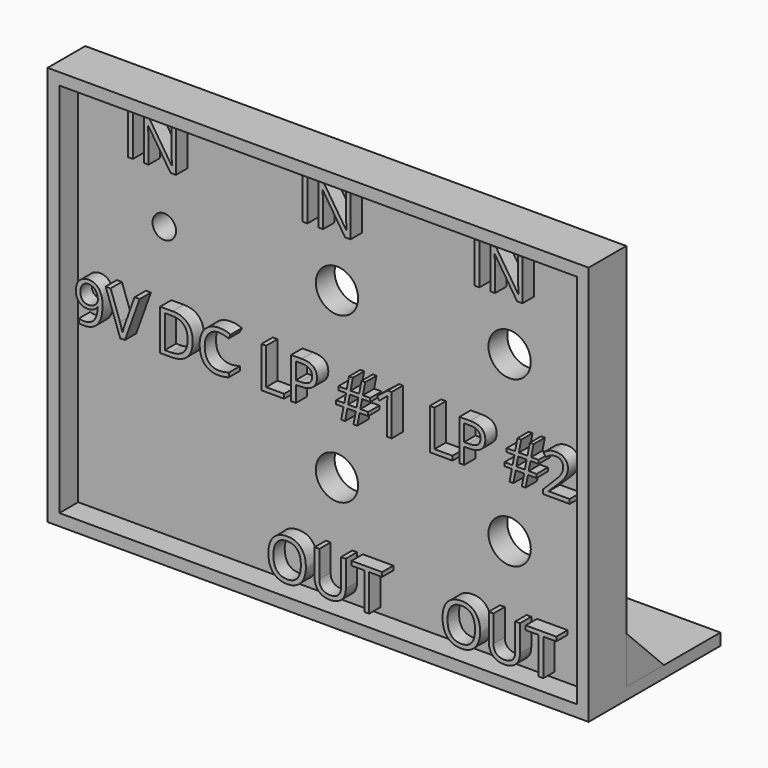
from build123d import *

# Parameters (mm, degrees)
F0_W          = 110
F0_H          = 80
F0_R          = 4.5
F0_R_2        = 2.5
F0_W_2        = 1.0082380031
F0_H_2        = 8.6754038348
F1_DEPTH      = 5
F2_DEPTH      = 10
F3_DEPTH      = 10
F3_DEPTH_BACK = 25
F0_TEXT_SIZE  = 12.1520211299
F4_DEPTH      = 8
F6_DEPTH      = 57.5


# Not quite as in the source:
# - Text() gives the source's letters only with a copy of the font that has no kerning and outlines rounded to 1/6400 em; it was checked with that copy


with BuildPart() as f1:
    # F0 (on Front) → F1 (new body)
    with BuildSketch(Plane.XZ):
        Rectangle(F0_W, F0_H)
        with BuildLine():
            add(Edge.make_bspline(
                [(-5.2528080414, -31.1302977692), (-4.2027974656, -32.3170185826), (-4.2027974656, -34.4056472143)],
                knots=[0, 0, 0, 1, 1, 1], degree=2))
            add(Edge.make_bspline(
                [(-4.2027974656, -34.4056472143), (-4.2027974656, -36.4885795861), (-5.256605548, -37.6819460362)],
                knots=[0, 0, 0, 1, 1, 1], degree=2))
            add(Edge.make_bspline(
                [(-5.256605548, -37.6819460362), (-6.3104136304, -38.8753124862), (-8.184483139, -38.8753124862)],
                knots=[0, 0, 0, 1, 1, 1], degree=2))
            add(Edge.make_bspline(
                [(-8.184483139, -38.8753124862), (-10.1003252203, -38.8753124862), (-11.1417914062, -37.7028323225)],
                knots=[0, 0, 0, 1, 1, 1], degree=2))
            add(Edge.make_bspline(
                [(-11.1417914062, -37.7028323225), (-12.1832575921, -36.5303521588), (-12.1832575921, -34.3942546945)],
                knots=[0, 0, 0, 1, 1, 1], degree=2))
            add(Edge.make_bspline(
                [(-12.1832575921, -34.3942546945), (-12.1832575921, -32.27524601), (-11.1389432762, -31.1094114829)],
                knots=[0, 0, 0, 1, 1, 1], degree=2))
            add(Edge.make_bspline(
                [(-11.1389432762, -31.1094114829), (-10.0946289604, -29.9435769557), (-8.1730906192, -29.9435769557)],
                knots=[0, 0, 0, 1, 1, 1], degree=2))
            add(Edge.make_bspline(
                [(-8.1730906192, -29.9435769557), (-6.3028186172, -29.9435769557), (-5.2528080414, -31.1302977692)],
                knots=[0, 0, 0, 1, 1, 1], degree=2))
        make_face(mode=Mode.SUBTRACT)
        with BuildLine():
            add(Edge.make_bspline(
                [(-47.7825725199, 2.592958442), (-47.4265562758, 1.7242788066), (-47.4265562758, 0.543254253)],
                knots=[0, 0, 0, 1, 1, 1], degree=2))
            add(Edge.make_bspline(
                [(-47.4265562758, 0.543254253), (-47.4265562758, -4.5492021018), (-51.3664693766, -4.5492021018)],
                knots=[0, 0, 0, 1, 1, 1], degree=2))
            add(Edge.make_bspline(
                [(-51.3664693766, -4.5492021018), (-52.055716825, -4.5492021018), (-52.458252525, -4.4295806438)],
                knots=[0, 0, 0, 1, 1, 1], degree=2))
            Line((-52.458252525, -4.4295806438), (-52.458252525, -3.580837918))
            add(Edge.make_bspline(
                [(-52.458252525, -3.580837918), (-51.9835641996, -3.7346369354), (-51.3797606497, -3.7346369354)],
                knots=[0, 0, 0, 1, 1, 1], degree=2))
            add(Edge.make_bspline(
                [(-51.3797606497, -3.7346369354), (-49.9556956735, -3.7346369354), (-49.228473159, -2.8536154035)],
                knots=[0, 0, 0, 1, 1, 1], degree=2))
            add(Edge.make_bspline(
                [(-49.228473159, -2.8536154035), (-48.5012506445, -1.9725938716), (-48.4366930323, -0.1516894554)],
                knots=[0, 0, 0, 1, 1, 1], degree=2))
            Line((-48.4366930323, -0.1516894554), (-48.5069469044, -0.1516894554))
            add(Edge.make_bspline(
                [(-48.5069469044, -0.1516894554), (-48.8335324723, -0.6434665605), (-49.3737277866, -0.9016970095)],
                knots=[0, 0, 0, 1, 1, 1], degree=2))
            add(Edge.make_bspline(
                [(-49.3737277866, -0.9016970095), (-49.9139231009, -1.1599274585), (-50.5898792762, -1.1599274585)],
                knots=[0, 0, 0, 1, 1, 1], degree=2))
            add(Edge.make_bspline(
                [(-50.5898792762, -1.1599274585), (-51.740523777, -1.1599274585), (-52.417429329, -0.4716293867)],
                knots=[0, 0, 0, 1, 1, 1], degree=2))
            add(Edge.make_bspline(
                [(-52.417429329, -0.4716293867), (-53.094334881, 0.2166686851), (-53.094334881, 1.4508583311)],
                knots=[0, 0, 0, 1, 1, 1], degree=2))
            add(Edge.make_bspline(
                [(-53.094334881, 1.4508583311), (-53.094334881, 2.8027706818), (-52.3376816903, 3.5860064187)],
                knots=[0, 0, 0, 1, 1, 1], degree=2))
            add(Edge.make_bspline(
                [(-52.3376816903, 3.5860064187), (-51.5810284996, 4.3692421556), (-50.3468388536, 4.3692421556)],
                knots=[0, 0, 0, 1, 1, 1], degree=2))
            add(Edge.make_bspline(
                [(-50.3468388536, 4.3692421556), (-49.4620198151, 4.3692421556), (-48.8003042895, 3.9154401165)],
                knots=[0, 0, 0, 1, 1, 1], degree=2))
            add(Edge.make_bspline(
                [(-48.8003042895, 3.9154401165), (-48.1385887639, 3.4616380775), (-47.7825725199, 2.592958442)],
                knots=[0, 0, 0, 1, 1, 1], degree=2))
        make_face(mode=Mode.SUBTRACT)
        with BuildLine():
            Line((-42.6094191498, -1.3327140089), (-40.627120703, 4.245823191))
            Line((-40.627120703, 4.245823191), (-39.5429325678, 4.245823191))
            Line((-39.5429325678, 4.245823191), (-42.6682805022, -4.4295806438))
            Line((-42.6682805022, -4.4295806438), (-43.6651259855, -4.4295806438))
            Line((-43.6651259855, -4.4295806438), (-46.7752838934, 4.245823191))
            Line((-46.7752838934, 4.245823191), (-45.7062857846, 4.245823191))
            Line((-45.7062857846, 4.245823191), (-43.712594818, -1.3668915684))
            add(Edge.make_bspline(
                [(-43.712594818, -1.3668915684), (-43.3689204704, -2.3352557522), (-43.1676526205, -3.2485560902)],
                knots=[0, 0, 0, 1, 1, 1], degree=2))
            add(Edge.make_bspline(
                [(-43.1676526205, -3.2485560902), (-42.9530934974, -2.2877869196), (-42.6094191498, -1.3327140089)],
                knots=[0, 0, 0, 1, 1, 1], degree=2))
        make_face(mode=Mode.SUBTRACT)
        with BuildLine():
            add(Edge.make_bspline(
                [(-29.3893492878, 3.1246093664), (-28.2681354632, 2.0033955419), (-28.2681354632, -0.0092829578)],
                knots=[0, 0, 0, 1, 1, 1], degree=2))
            add(Edge.make_bspline(
                [(-28.2681354632, -0.0092829578), (-28.2681354632, -2.1567729418), (-29.4339699904, -3.2931767928)],
                knots=[0, 0, 0, 1, 1, 1], degree=2))
            add(Edge.make_bspline(
                [(-29.4339699904, -3.2931767928), (-30.5998045175, -4.4295806438), (-32.7890670742, -4.4295806438)],
                knots=[0, 0, 0, 1, 1, 1], degree=2))
            Line((-32.7890670742, -4.4295806438), (-35.192888754, -4.4295806438))
            Line((-35.192888754, -4.4295806438), (-35.192888754, 4.245823191))
            Line((-35.192888754, 4.245823191), (-32.5346341318, 4.245823191))
            add(Edge.make_bspline(
                [(-32.5346341318, 4.245823191), (-30.5105631123, 4.245823191), (-29.3893492878, 3.1246093664)],
                knots=[0, 0, 0, 1, 1, 1], degree=2))
        make_face(mode=Mode.SUBTRACT)
        with BuildLine():
            add(Edge.make_bspline(
                [(-20.6484384641, 3.0059372851), (-21.6338914276, 3.4673343374), (-22.6193443911, 3.4673343374)],
                knots=[0, 0, 0, 1, 1, 1], degree=2))
            add(Edge.make_bspline(
                [(-22.6193443911, 3.4673343374), (-24.0491056272, 3.4673343374), (-24.8769620666, 2.5151095566)],
                knots=[0, 0, 0, 1, 1, 1], degree=2))
            add(Edge.make_bspline(
                [(-24.8769620666, 2.5151095566), (-25.7048185061, 1.5628847759), (-25.7048185061, -0.092828103)],
                knots=[0, 0, 0, 1, 1, 1], degree=2))
            add(Edge.make_bspline(
                [(-25.7048185061, -0.092828103), (-25.7048185061, -1.7941110612), (-24.9063927428, -2.7235508023)],
                knots=[0, 0, 0, 1, 1, 1], degree=2))
            add(Edge.make_bspline(
                [(-24.9063927428, -2.7235508023), (-24.1079669795, -3.6529905434), (-22.6307369109, -3.6529905434)],
                knots=[0, 0, 0, 1, 1, 1], degree=2))
            add(Edge.make_bspline(
                [(-22.6307369109, -3.6529905434), (-21.7231328328, -3.6529905434), (-20.5591970589, -3.3264049756)],
                knots=[0, 0, 0, 1, 1, 1], degree=2))
            Line((-20.5591970589, -3.3264049756), (-20.5591970589, -4.2093252608))
            add(Edge.make_bspline(
                [(-20.5591970589, -4.2093252608), (-21.4611048771, -4.5492021018), (-22.7845359283, -4.5492021018)],
                knots=[0, 0, 0, 1, 1, 1], degree=2))
            add(Edge.make_bspline(
                [(-22.7845359283, -4.5492021018), (-24.7003780096, -4.5492021018), (-25.7418441955, -3.3852663279)],
                knots=[0, 0, 0, 1, 1, 1], degree=2))
            add(Edge.make_bspline(
                [(-25.7418441955, -3.3852663279), (-26.7833103814, -2.2213305541), (-26.7833103814, -0.0795368299)],
                knots=[0, 0, 0, 1, 1, 1], degree=2))
            add(Edge.make_bspline(
                [(-26.7833103814, -0.0795368299), (-26.7833103814, 1.260983001), (-26.2820395098, 2.2692210041)],
                knots=[0, 0, 0, 1, 1, 1], degree=2))
            add(Edge.make_bspline(
                [(-26.2820395098, 2.2692210041), (-25.7807686382, 3.2774590072), (-24.8342401173, 3.8233505814)],
                knots=[0, 0, 0, 1, 1, 1], degree=2))
            add(Edge.make_bspline(
                [(-24.8342401173, 3.8233505814), (-23.8877115965, 4.3692421556), (-22.606053118, 4.3692421556)],
                knots=[0, 0, 0, 1, 1, 1], degree=2))
            add(Edge.make_bspline(
                [(-22.606053118, 4.3692421556), (-21.2427482475, 4.3692421556), (-20.2212189712, 3.8717687906)],
                knots=[0, 0, 0, 1, 1, 1], degree=2))
            Line((-20.2212189712, 3.8717687906), (-20.6484384641, 3.0059372851))
        make_face(mode=Mode.SUBTRACT)
        Polygon((-8.8162453418, -4.4000898488), (-13.6523700009, -4.4000898488), (-13.6523700009, 4.275313986), (-12.6441319978, 4.275313986), (-12.6441319978, -3.4867895107), (-8.8162453418, -3.4867895107), align=None, mode=Mode.SUBTRACT)
        with BuildLine():
            add(Edge.make_bspline(
                [(-5.0946888708, 4.275313986), (-1.8440232185, 4.275313986), (-1.8440232185, 1.7480733416)],
                knots=[0, 0, 0, 1, 1, 1], degree=2))
            add(Edge.make_bspline(
                [(-1.8440232185, 1.7480733416), (-1.8440232185, 0.4303385504), (-2.7430829068, -0.2788458078)],
                knots=[0, 0, 0, 1, 1, 1], degree=2))
            add(Edge.make_bspline(
                [(-2.7430829068, -0.2788458078), (-3.6421425951, -0.9880301659), (-5.3149442538, -0.9880301659)],
                knots=[0, 0, 0, 1, 1, 1], degree=2))
            Line((-5.3149442538, -0.9880301659), (-6.33647353, -0.9880301659))
            Line((-6.33647353, -0.9880301659), (-6.33647353, -4.4000898488))
            Line((-6.33647353, -4.4000898488), (-7.3447115331, -4.4000898488))
            Line((-7.3447115331, -4.4000898488), (-7.3447115331, 4.275313986))
            Line((-7.3447115331, 4.275313986), (-5.0946888708, 4.275313986))
        make_face(mode=Mode.SUBTRACT)
        with BuildLine():
            Line((3.2725942826, -30.0802871934), (4.2808322857, -30.0802871934))
            Line((4.2808322857, -30.0802871934), (4.2808322857, -35.6930019528))
            add(Edge.make_bspline(
                [(4.2808322857, -35.6930019528), (4.2808322857, -37.1778270346), (3.3846207274, -38.0265697604)],
                knots=[0, 0, 0, 1, 1, 1], degree=2))
            add(Edge.make_bspline(
                [(3.3846207274, -38.0265697604), (2.488409169, -38.8753124862), (0.9219376952, -38.8753124862)],
                knots=[0, 0, 0, 1, 1, 1], degree=2))
            add(Edge.make_bspline(
                [(0.9219376952, -38.8753124862), (-0.6445337785, -38.8753124862), (-1.5018208942, -38.0199241238)],
                knots=[0, 0, 0, 1, 1, 1], degree=2))
            add(Edge.make_bspline(
                [(-1.5018208942, -38.0199241238), (-2.3591080098, -37.1645357615), (-2.3591080098, -35.6702169132)],
                knots=[0, 0, 0, 1, 1, 1], degree=2))
            Line((-2.3591080098, -35.6702169132), (-2.3591080098, -30.0802871934))
            Line((-2.3591080098, -30.0802871934), (-1.3489712534, -30.0802871934))
            Line((-1.3489712534, -30.0802871934), (-1.3489712534, -35.7404707853))
            add(Edge.make_bspline(
                [(-1.3489712534, -35.7404707853), (-1.3489712534, -36.8265576738), (-0.7556108467, -37.4085255607)],
                knots=[0, 0, 0, 1, 1, 1], degree=2))
            add(Edge.make_bspline(
                [(-0.7556108467, -37.4085255607), (-0.1622504399, -37.9904934477), (0.9883940608, -37.9904934477)],
                knots=[0, 0, 0, 1, 1, 1], degree=2))
            add(Edge.make_bspline(
                [(0.9883940608, -37.9904934477), (2.0858734691, -37.9904934477), (2.6792338758, -37.4056774308)],
                knots=[0, 0, 0, 1, 1, 1], degree=2))
            add(Edge.make_bspline(
                [(2.6792338758, -37.4056774308), (3.2725942826, -36.8208614139), (3.2725942826, -35.7290782655)],
                knots=[0, 0, 0, 1, 1, 1], degree=2))
            Line((3.2725942826, -35.7290782655), (3.2725942826, -30.0802871934))
        make_face(mode=Mode.SUBTRACT)
        Polygon((9.2460721692, -30.9764987517), (9.2460721692, -38.7556910282), (8.2378341661, -38.7556910282), (8.2378341661, -30.9764987517), (5.4903381388, -30.9764987517), (5.4903381388, -30.0802871934), (11.9935681966, -30.0802871934), (11.9935681966, -30.9764987517), align=None, mode=Mode.SUBTRACT)
        with BuildLine():
            add(Edge.make_bspline(
                [(31.7720284802, -31.1662295911), (32.8220390559, -32.3529504046), (32.8220390559, -34.4415790363)],
                knots=[0, 0, 0, 1, 1, 1], degree=2))
            add(Edge.make_bspline(
                [(32.8220390559, -34.4415790363), (32.8220390559, -36.5245114081), (31.7682309736, -37.7178778581)],
                knots=[0, 0, 0, 1, 1, 1], degree=2))
            add(Edge.make_bspline(
                [(31.7682309736, -37.7178778581), (30.7144228912, -38.9112443081), (28.8403533826, -38.9112443081)],
                knots=[0, 0, 0, 1, 1, 1], degree=2))
            add(Edge.make_bspline(
                [(28.8403533826, -38.9112443081), (26.9245113013, -38.9112443081), (25.8830451154, -37.7387641444)],
                knots=[0, 0, 0, 1, 1, 1], degree=2))
            add(Edge.make_bspline(
                [(25.8830451154, -37.7387641444), (24.8415789295, -36.5662839807), (24.8415789295, -34.4301865165)],
                knots=[0, 0, 0, 1, 1, 1], degree=2))
            add(Edge.make_bspline(
                [(24.8415789295, -34.4301865165), (24.8415789295, -32.3111778319), (25.8858932454, -31.1453433048)],
                knots=[0, 0, 0, 1, 1, 1], degree=2))
            add(Edge.make_bspline(
                [(25.8858932454, -31.1453433048), (26.9302075612, -29.9795087776), (28.8517459024, -29.9795087776)],
                knots=[0, 0, 0, 1, 1, 1], degree=2))
            add(Edge.make_bspline(
                [(28.8517459024, -29.9795087776), (30.7220179044, -29.9795087776), (31.7720284802, -31.1662295911)],
                knots=[0, 0, 0, 1, 1, 1], degree=2))
        make_face(mode=Mode.SUBTRACT)
        with BuildLine():
            Line((40.2974308042, -30.1162190153), (41.3056688073, -30.1162190153))
            Line((41.3056688073, -30.1162190153), (41.3056688073, -35.7289337747))
            add(Edge.make_bspline(
                [(41.3056688073, -35.7289337747), (41.3056688073, -37.2137588565), (40.4094572489, -38.0625015823)],
                knots=[0, 0, 0, 1, 1, 1], degree=2))
            add(Edge.make_bspline(
                [(40.4094572489, -38.0625015823), (39.5132456906, -38.9112443081), (37.9467742168, -38.9112443081)],
                knots=[0, 0, 0, 1, 1, 1], degree=2))
            add(Edge.make_bspline(
                [(37.9467742168, -38.9112443081), (36.3803027431, -38.9112443081), (35.5230156274, -38.0558559458)],
                knots=[0, 0, 0, 1, 1, 1], degree=2))
            add(Edge.make_bspline(
                [(35.5230156274, -38.0558559458), (34.6657285118, -37.2004675834), (34.6657285118, -35.7061487351)],
                knots=[0, 0, 0, 1, 1, 1], degree=2))
            Line((34.6657285118, -35.7061487351), (34.6657285118, -30.1162190153))
            Line((34.6657285118, -30.1162190153), (35.6758652682, -30.1162190153))
            Line((35.6758652682, -30.1162190153), (35.6758652682, -35.7764026072))
            add(Edge.make_bspline(
                [(35.6758652682, -35.7764026072), (35.6758652682, -36.8624894957), (36.2692256749, -37.4444573827)],
                knots=[0, 0, 0, 1, 1, 1], degree=2))
            add(Edge.make_bspline(
                [(36.2692256749, -37.4444573827), (36.8625860816, -38.0264252696), (38.0132305824, -38.0264252696)],
                knots=[0, 0, 0, 1, 1, 1], degree=2))
            add(Edge.make_bspline(
                [(38.0132305824, -38.0264252696), (39.1107099907, -38.0264252696), (39.7040703974, -37.4416092527)],
                knots=[0, 0, 0, 1, 1, 1], degree=2))
            add(Edge.make_bspline(
                [(39.7040703974, -37.4416092527), (40.2974308042, -36.8567932358), (40.2974308042, -35.7650100874)],
                knots=[0, 0, 0, 1, 1, 1], degree=2))
            Line((40.2974308042, -35.7650100874), (40.2974308042, -30.1162190153))
        make_face(mode=Mode.SUBTRACT)
        Polygon((46.2709086908, -31.0124305737), (46.2709086908, -38.7916228501), (45.2626706877, -38.7916228501), (45.2626706877, -31.0124305737), (42.5151746604, -31.0124305737), (42.5151746604, -30.1162190153), (49.0184047182, -30.1162190153), (49.0184047182, -31.0124305737), align=None, mode=Mode.SUBTRACT)
        with Locations((0, -17.5)):
            Circle(F0_R, mode=Mode.SUBTRACT)
        Polygon((9.4725464587, 0.9335081753), (7.7579722274, 0.9335081753), (7.364930294, -1.082967831), (9.0453269659, -1.082967831), (9.0453269659, -1.8481654115), (7.2225237964, -1.8481654115), (6.7250504314, -4.4000898488), (5.9123840183, -4.4000898488), (6.4098573833, -1.8481654115), (4.6117380067, -1.8481654115), (4.1256571615, -4.4000898488), (3.3186870084, -4.4000898488), (3.7933753338, -1.8481654115), (2.2382963798, -1.8481654115), (2.2382963798, -1.082967831), (3.9414780913, -1.082967831), (4.3459125445, 0.9335081753), (2.7015921854, 0.9335081753), (2.7015921854, 1.687313236), (4.4769265223, 1.687313236), (4.9630073675, 4.275313986), (5.7870663004, 4.275313986), (5.3009854552, 1.687313236), (7.1104973516, 1.687313236), (7.6098694699, 4.275313986), (8.4035483499, 4.275313986), (7.9060749849, 1.687313236), (9.4725464587, 1.687313236), align=None, mode=Mode.SUBTRACT)
        with BuildLine():
            Line((14.0276556291, 4.275313986), (14.0276556291, -4.4000898488))
            Line((14.0276556291, -4.4000898488), (13.0668864585, -4.4000898488))
            Line((13.0668864585, -4.4000898488), (13.0668864585, 1.7822509011))
            add(Edge.make_bspline(
                [(13.0668864585, 1.7822509011), (13.0668864585, 2.5550434948), (13.1143552911, 3.24239219)],
                knots=[0, 0, 0, 1, 1, 1], degree=2))
            add(Edge.make_bspline(
                [(13.1143552911, 3.24239219), (12.9909363265, 3.1170744721), (12.8361879324, 2.981313611)],
                knots=[0, 0, 0, 1, 1, 1], degree=2))
            add(Edge.make_bspline(
                [(12.8361879324, 2.981313611), (12.6814395383, 2.8455527499), (11.4244648527, 1.8240234737)],
                knots=[0, 0, 0, 1, 1, 1], degree=2))
            Line((11.4244648527, 1.8240234737), (10.9023076948, 2.4999796491))
            Line((10.9023076948, 2.4999796491), (13.1979004364, 4.275313986))
            Line((13.1979004364, 4.275313986), (14.0276556291, 4.275313986))
        make_face(mode=Mode.SUBTRACT)
        Polygon((26.9632575995, -4.3550701812), (22.1271329404, -4.3550701812), (22.1271329404, 4.3203336536), (23.1353709435, 4.3203336536), (23.1353709435, -3.4417698431), (26.9632575995, -3.4417698431), align=None, mode=Mode.SUBTRACT)
        with Locations((36.7, -17.5)):
            Circle(F0_R, mode=Mode.SUBTRACT)
        with BuildLine():
            add(Edge.make_bspline(
                [(30.6848140705, 4.3203336536), (33.9354797228, 4.3203336536), (33.9354797228, 1.7930930092)],
                knots=[0, 0, 0, 1, 1, 1], degree=2))
            add(Edge.make_bspline(
                [(33.9354797228, 1.7930930092), (33.9354797228, 0.475358218), (33.0364200345, -0.2338261402)],
                knots=[0, 0, 0, 1, 1, 1], degree=2))
            add(Edge.make_bspline(
                [(33.0364200345, -0.2338261402), (32.1373603462, -0.9430104983), (30.4645586875, -0.9430104983)],
                knots=[0, 0, 0, 1, 1, 1], degree=2))
            Line((30.4645586875, -0.9430104983), (29.4430294113, -0.9430104983))
            Line((29.4430294113, -0.9430104983), (29.4430294113, -4.3550701812))
            Line((29.4430294113, -4.3550701812), (28.4347914082, -4.3550701812))
            Line((28.4347914082, -4.3550701812), (28.4347914082, 4.3203336536))
            Line((28.4347914082, 4.3203336536), (30.6848140705, 4.3203336536))
        make_face(mode=Mode.SUBTRACT)
        Polygon((45.2520494, 0.9785278429), (43.5374751687, 0.9785278429), (43.1444332353, -1.0379481634), (44.8248299072, -1.0379481634), (44.8248299072, -1.8031457439), (43.0020267377, -1.8031457439), (42.5045533727, -4.3550701812), (41.6918869596, -4.3550701812), (42.1893603246, -1.8031457439), (40.391240948, -1.8031457439), (39.9051601028, -4.3550701812), (39.0981899497, -4.3550701812), (39.5728782751, -1.8031457439), (38.0177993211, -1.8031457439), (38.0177993211, -1.0379481634), (39.7209810326, -1.0379481634), (40.1254154858, 0.9785278429), (38.4810951267, 0.9785278429), (38.4810951267, 1.7323329036), (40.2564294636, 1.7323329036), (40.7425103088, 4.3203336536), (41.5665692417, 4.3203336536), (41.0804883965, 1.7323329036), (42.8900002929, 1.7323329036), (43.3893724112, 4.3203336536), (44.1830512912, 4.3203336536), (43.6855779262, 1.7323329036), (45.2520494, 1.7323329036), align=None, mode=Mode.SUBTRACT)
        with Locations((-36.7, 17.5)):
            Circle(F0_R_2, mode=Mode.SUBTRACT)
        with Locations((-41.4737182534, 34.3377019174)):
            Rectangle(F0_W_2, F0_H_2, mode=Mode.SUBTRACT)
        with BuildLine():
            Line((-31.8138108317, 38.6754038348), (-31.8138108317, 30))
            Line((-31.8138108317, 30), (-32.9644553325, 30))
            Line((-32.9644553325, 30), (-37.7056423264, 37.2798201581))
            Line((-37.7056423264, 37.2798201581), (-37.753111159, 37.2798201581))
            add(Edge.make_bspline(
                [(-37.753111159, 37.2798201581), (-37.6581734939, 35.9981616796), (-37.6581734939, 34.9310623241)],
                knots=[0, 0, 0, 1, 1, 1], degree=2))
            Line((-37.6581734939, 34.9310623241), (-37.6581734939, 30))
            Line((-37.6581734939, 30), (-38.5904613649, 30))
            Line((-38.5904613649, 30), (-38.5904613649, 38.6754038348))
            Line((-38.5904613649, 38.6754038348), (-37.451209384, 38.6754038348))
            Line((-37.451209384, 38.6754038348), (-32.7214149099, 31.4240649762))
            Line((-32.7214149099, 31.4240649762), (-32.6739460773, 31.4240649762))
            add(Edge.make_bspline(
                [(-32.6739460773, 31.4240649762), (-32.6853385971, 31.5835602535), (-32.7271111698, 32.4531892656)],
                knots=[0, 0, 0, 1, 1, 1], degree=2))
            add(Edge.make_bspline(
                [(-32.7271111698, 32.4531892656), (-32.7688837424, 33.3228182777), (-32.7574912226, 33.6968726781)],
                knots=[0, 0, 0, 1, 1, 1], degree=2))
            Line((-32.7574912226, 33.6968726781), (-32.7574912226, 38.6754038348))
            Line((-32.7574912226, 38.6754038348), (-31.8138108317, 38.6754038348))
        make_face(mode=Mode.SUBTRACT)
        with Locations((-4.3756769834, 34.3386251188)):
            Rectangle(F0_W_2, F0_H_2, mode=Mode.SUBTRACT)
        with Locations((0, 17.5)):
            Circle(F0_R, mode=Mode.SUBTRACT)
        with BuildLine():
            Line((51.8616096427, -3.4417698431), (51.8616096427, -4.3550701812))
            Line((51.8616096427, -4.3550701812), (46.1596534781, -4.3550701812))
            Line((46.1596534781, -4.3550701812), (46.1596534781, -3.5063274554))
            Line((46.1596534781, -3.5063274554), (48.4438536999, -1.2107347138))
            add(Edge.make_bspline(
                [(48.4438536999, -1.2107347138), (49.4881680158, -0.1531291249), (49.8204498435, 0.2978247843)],
                knots=[0, 0, 0, 1, 1, 1], degree=2))
            add(Edge.make_bspline(
                [(49.8204498435, 0.2978247843), (50.1527316713, 0.7487786934), (50.3188725852, 1.1759981862)],
                knots=[0, 0, 0, 1, 1, 1], degree=2))
            add(Edge.make_bspline(
                [(50.3188725852, 1.1759981862), (50.4850134991, 1.6032176791), (50.4850134991, 2.0949947842)],
                knots=[0, 0, 0, 1, 1, 1], degree=2))
            add(Edge.make_bspline(
                [(50.4850134991, 2.0949947842), (50.4850134991, 2.7899384925), (50.0634902661, 3.1962716991)],
                knots=[0, 0, 0, 1, 1, 1], degree=2))
            add(Edge.make_bspline(
                [(50.0634902661, 3.1962716991), (49.6419670332, 3.6026049056), (48.8938582324, 3.6026049056)],
                knots=[0, 0, 0, 1, 1, 1], degree=2))
            add(Edge.make_bspline(
                [(48.8938582324, 3.6026049056), (48.3546122947, 3.6026049056), (47.8704302028, 3.4241220953)],
                knots=[0, 0, 0, 1, 1, 1], degree=2))
            add(Edge.make_bspline(
                [(47.8704302028, 3.4241220953), (47.3862481109, 3.2456392849), (46.7938370809, 2.7766472194)],
                knots=[0, 0, 0, 1, 1, 1], degree=2))
            Line((46.7938370809, 2.7766472194), (46.2716799229, 3.4469071349))
            add(Edge.make_bspline(
                [(46.2716799229, 3.4469071349), (47.4697932562, 4.4437526182), (48.8824657126, 4.4437526182)],
                knots=[0, 0, 0, 1, 1, 1], degree=2))
            add(Edge.make_bspline(
                [(48.8824657126, 4.4437526182), (50.1052628388, 4.4437526182), (50.7992571705, 3.8181134053)],
                knots=[0, 0, 0, 1, 1, 1], degree=2))
            add(Edge.make_bspline(
                [(50.7992571705, 3.8181134053), (51.4932515022, 3.1924741925), (51.4932515022, 2.1367673568)],
                knots=[0, 0, 0, 1, 1, 1], degree=2))
            add(Edge.make_bspline(
                [(51.4932515022, 2.1367673568), (51.4932515022, 1.3108096706), (51.0299556966, 0.5038395175)],
                knots=[0, 0, 0, 1, 1, 1], degree=2))
            add(Edge.make_bspline(
                [(51.0299556966, 0.5038395175), (50.566659891, -0.3031306357), (49.2982926856, -1.5373202817)],
                knots=[0, 0, 0, 1, 1, 1], degree=2))
            Line((49.2982926856, -1.5373202817), (47.3995393841, -3.3943010106))
            Line((47.3995393841, -3.3943010106), (47.3995393841, -3.4417698431))
            Line((47.3995393841, -3.4417698431), (51.8616096427, -3.4417698431))
        make_face(mode=Mode.SUBTRACT)
        with Locations((36.7, 17.5)):
            Circle(F0_R, mode=Mode.SUBTRACT)
        with BuildLine():
            Line((5.2842304382, 38.6763270362), (5.2842304382, 30.0009232014))
            Line((5.2842304382, 30.0009232014), (4.1335859375, 30.0009232014))
            Line((4.1335859375, 30.0009232014), (-0.6076010565, 37.2807433596))
            Line((-0.6076010565, 37.2807433596), (-0.655069889, 37.2807433596))
            add(Edge.make_bspline(
                [(-0.655069889, 37.2807433596), (-0.560132224, 35.999084881), (-0.560132224, 34.9319855256)],
                knots=[0, 0, 0, 1, 1, 1], degree=2))
            Line((-0.560132224, 34.9319855256), (-0.560132224, 30.0009232014))
            Line((-0.560132224, 30.0009232014), (-1.492420095, 30.0009232014))
            Line((-1.492420095, 30.0009232014), (-1.492420095, 38.6763270362))
            Line((-1.492420095, 38.6763270362), (-0.3531681141, 38.6763270362))
            Line((-0.3531681141, 38.6763270362), (4.3766263601, 31.4249881776))
            Line((4.3766263601, 31.4249881776), (4.4240951926, 31.4249881776))
            add(Edge.make_bspline(
                [(4.4240951926, 31.4249881776), (4.4127026728, 31.5844834549), (4.3709301002, 32.454112467)],
                knots=[0, 0, 0, 1, 1, 1], degree=2))
            add(Edge.make_bspline(
                [(4.3709301002, 32.454112467), (4.3291575275, 33.3237414792), (4.3405500473, 33.6977958796)],
                knots=[0, 0, 0, 1, 1, 1], degree=2))
            Line((4.3405500473, 33.6977958796), (4.3405500473, 38.6763270362))
            Line((4.3405500473, 38.6763270362), (5.2842304382, 38.6763270362))
        make_face(mode=Mode.SUBTRACT)
        with Locations((32.188025992, 34.2669188685)):
            Rectangle(F0_W_2, F0_H_2, mode=Mode.SUBTRACT)
        with BuildLine():
            Line((41.8479334136, 38.6046207859), (41.8479334136, 29.9292169511))
            Line((41.8479334136, 29.9292169511), (40.6972889129, 29.9292169511))
            Line((40.6972889129, 29.9292169511), (35.9561019189, 37.2090371093))
            Line((35.9561019189, 37.2090371093), (35.9086330864, 37.2090371093))
            add(Edge.make_bspline(
                [(35.9086330864, 37.2090371093), (36.0035707514, 35.9273786307), (36.0035707514, 34.8602792753)],
                knots=[0, 0, 0, 1, 1, 1], degree=2))
            Line((36.0035707514, 34.8602792753), (36.0035707514, 29.9292169511))
            Line((36.0035707514, 29.9292169511), (35.0712828804, 29.9292169511))
            Line((35.0712828804, 29.9292169511), (35.0712828804, 38.6046207859))
            Line((35.0712828804, 38.6046207859), (36.2105348613, 38.6046207859))
            Line((36.2105348613, 38.6046207859), (40.9403293355, 31.3532819273))
            Line((40.9403293355, 31.3532819273), (40.987798168, 31.3532819273))
            add(Edge.make_bspline(
                [(40.987798168, 31.3532819273), (40.9764056482, 31.5127772046), (40.9346330756, 32.3824062167)],
                knots=[0, 0, 0, 1, 1, 1], degree=2))
            add(Edge.make_bspline(
                [(40.9346330756, 32.3824062167), (40.8928605029, 33.2520352288), (40.9042530227, 33.6260896293)],
                knots=[0, 0, 0, 1, 1, 1], degree=2))
            Line((40.9042530227, 33.6260896293), (40.9042530227, 38.6046207859))
            Line((40.9042530227, 38.6046207859), (41.8479334136, 38.6046207859))
        make_face(mode=Mode.SUBTRACT)
    extrude(amount=F1_DEPTH)

    # F0 (on Front) → F2 (join)
    with BuildSketch(Plane.XZ):
        Polygon((-55, -40), (-55, 40), (55, 40), (55, -40), (57.5, -40), (57.5, 42.5), (-57.5, 42.5), (-57.5, -40), align=None)
    extrude(amount=F2_DEPTH)

    # F0 (on Front) → F3 (join, two sides)
    with BuildSketch(Plane.XZ) as f3_sk:
        Polygon((55, -40), (-55, -40), (-57.5, -40), (-57.5, -42.5), (57.5, -42.5), (57.5, -40), align=None)
    extrude(amount=F3_DEPTH)
    extrude(f3_sk.sketch, amount=-F3_DEPTH_BACK)

    # F0 (on Front) → F4 (join)
    with BuildSketch(Plane.XZ):
        with Locations((30.491489917, 29.9292169511)):
            Text('IN', F0_TEXT_SIZE, font='Open Sans', text_align=(TextAlign.LEFT, TextAlign.BOTTOM))
        with Locations((-6.0722130584, 30.0009232014)):
            Text('IN', F0_TEXT_SIZE, font='Open Sans', text_align=(TextAlign.LEFT, TextAlign.BOTTOM))
        with Locations((-43.1702543283, 30)):
            Text('IN', F0_TEXT_SIZE, font='Open Sans', text_align=(TextAlign.LEFT, TextAlign.BOTTOM))
        with Locations((-53.7228222238, -4.4295806438)):
            Text('9V DC', F0_TEXT_SIZE, font='Open Sans', text_align=(TextAlign.LEFT, TextAlign.BOTTOM))
        with Locations((-14.8447870743, -4.4000898488)):
            Text('LP #1', F0_TEXT_SIZE, font='Open Sans', text_align=(TextAlign.LEFT, TextAlign.BOTTOM))
        with Locations((20.934715867, -4.3550701812)):
            Text('LP #2', F0_TEXT_SIZE, font='Open Sans', text_align=(TextAlign.LEFT, TextAlign.BOTTOM))
        with Locations((24.0991663886, -38.7916228501)):
            Text('OUT', F0_TEXT_SIZE, font='Open Sans', text_align=(TextAlign.LEFT, TextAlign.BOTTOM))
        with Locations((-12.925670133, -38.7556910282)):
            Text('OUT', F0_TEXT_SIZE, font='Open Sans', text_align=(TextAlign.LEFT, TextAlign.BOTTOM))
    extrude(amount=F4_DEPTH)


with BuildPart() as f1b:
    # F0 (on Front) → F1, piece 2 (new body)
    with BuildSketch(Plane.XZ):
        with BuildLine():
            add(Edge.make_bspline(
                [(-49.3471452404, 3.2252432914), (-49.7829091231, 3.528094443), (-50.3468388536, 3.528094443)],
                knots=[0, 0, 0, 1, 1, 1], degree=2))
            add(Edge.make_bspline(
                [(-50.3468388536, 3.528094443), (-51.1955815794, 3.528094443), (-51.6579280084, 2.9822028688)],
                knots=[0, 0, 0, 1, 1, 1], degree=2))
            add(Edge.make_bspline(
                [(-51.6579280084, 2.9822028688), (-52.1202744373, 2.4363112946), (-52.1202744373, 1.4622508509)],
                knots=[0, 0, 0, 1, 1, 1], degree=2))
            add(Edge.make_bspline(
                [(-52.1202744373, 1.4622508509), (-52.1202744373, 0.6078118652), (-51.6930549444, 0.1188828901)],
                knots=[0, 0, 0, 1, 1, 1], degree=2))
            add(Edge.make_bspline(
                [(-51.6930549444, 0.1188828901), (-51.2658354516, -0.3700460851), (-50.3943076862, -0.3700460851)],
                knots=[0, 0, 0, 1, 1, 1], degree=2))
            add(Edge.make_bspline(
                [(-50.3943076862, -0.3700460851), (-49.8531629952, -0.3700460851), (-49.3993609562, -0.1507400787)],
                knots=[0, 0, 0, 1, 1, 1], degree=2))
            add(Edge.make_bspline(
                [(-49.3993609562, -0.1507400787), (-48.9455589171, 0.0685659276), (-48.6844803381, 0.4483165879)],
                knots=[0, 0, 0, 1, 1, 1], degree=2))
            add(Edge.make_bspline(
                [(-48.6844803381, 0.4483165879), (-48.4234017592, 0.8280672482), (-48.4234017592, 1.2438942213)],
                knots=[0, 0, 0, 1, 1, 1], degree=2))
            add(Edge.make_bspline(
                [(-48.4234017592, 1.2438942213), (-48.4234017592, 1.8666853042), (-48.6673915584, 2.394538722)],
                knots=[0, 0, 0, 1, 1, 1], degree=2))
            add(Edge.make_bspline(
                [(-48.6673915584, 2.394538722), (-48.9113813577, 2.9223921398), (-49.3471452404, 3.2252432914)],
                knots=[0, 0, 0, 1, 1, 1], degree=2))
        make_face()
    extrude(amount=F1_DEPTH)


with BuildPart() as f1c:
    # F0 (on Front) → F1, piece 3 (new body)
    with BuildSketch(Plane.XZ):
        with BuildLine():
            add(Edge.make_bspline(
                [(-30.2437882735, -2.6703857099), (-29.3352348187, -1.7827185414), (-29.3352348187, -0.0453592705)],
                knots=[0, 0, 0, 1, 1, 1], degree=2))
            add(Edge.make_bspline(
                [(-29.3352348187, -0.0453592705), (-29.3352348187, 1.6521261811), (-30.1868256744, 2.5122614267)],
                knots=[0, 0, 0, 1, 1, 1], degree=2))
            add(Edge.make_bspline(
                [(-30.1868256744, 2.5122614267), (-31.0384165302, 3.3723966723), (-32.718813202, 3.3723966723)],
                knots=[0, 0, 0, 1, 1, 1], degree=2))
            Line((-32.718813202, 3.3723966723), (-34.1846507508, 3.3723966723))
            Line((-34.1846507508, 3.3723966723), (-34.1846507508, -3.5580528784))
            Line((-34.1846507508, -3.5580528784), (-32.9561573647, -3.5580528784))
            add(Edge.make_bspline(
                [(-32.9561573647, -3.5580528784), (-31.1523417283, -3.5580528784), (-30.2437882735, -2.6703857099)],
                knots=[0, 0, 0, 1, 1, 1], degree=2))
        make_face()
    extrude(amount=F1_DEPTH)


with BuildPart() as f1d:
    # F0 (on Front) → F1, piece 4 (new body)
    with BuildSketch(Plane.XZ):
        with BuildLine():
            add(Edge.make_bspline(
                [(-10.3652013058, -31.7568863587), (-11.1161582366, -32.6682879434), (-11.1161582366, -34.4056472143)],
                knots=[0, 0, 0, 1, 1, 1], degree=2))
            add(Edge.make_bspline(
                [(-11.1161582366, -34.4056472143), (-11.1161582366, -36.1676902782), (-10.3652013058, -37.0790918629)],
                knots=[0, 0, 0, 1, 1, 1], degree=2))
            add(Edge.make_bspline(
                [(-10.3652013058, -37.0790918629), (-9.6142443751, -37.9904934477), (-8.184483139, -37.9904934477)],
                knots=[0, 0, 0, 1, 1, 1], degree=2))
            add(Edge.make_bspline(
                [(-8.184483139, -37.9904934477), (-6.7433293831, -37.9904934477), (-6.0075624788, -37.0828893695)],
                knots=[0, 0, 0, 1, 1, 1], degree=2))
            add(Edge.make_bspline(
                [(-6.0075624788, -37.0828893695), (-5.2717955744, -36.1752852914), (-5.2717955744, -34.4056472143)],
                knots=[0, 0, 0, 1, 1, 1], degree=2))
            add(Edge.make_bspline(
                [(-5.2717955744, -34.4056472143), (-5.2717955744, -32.6549966703), (-6.0047143488, -31.7502407221)],
                knots=[0, 0, 0, 1, 1, 1], degree=2))
            add(Edge.make_bspline(
                [(-6.0047143488, -31.7502407221), (-6.7376331232, -30.8454847739), (-8.1730906192, -30.8454847739)],
                knots=[0, 0, 0, 1, 1, 1], degree=2))
            add(Edge.make_bspline(
                [(-8.1730906192, -30.8454847739), (-9.6142443751, -30.8454847739), (-10.3652013058, -31.7568863587)],
                knots=[0, 0, 0, 1, 1, 1], degree=2))
        make_face()
    extrude(amount=F1_DEPTH)


with BuildPart() as f1e:
    # F0 (on Front) → F1, piece 5 (new body)
    with BuildSketch(Plane.XZ):
        with BuildLine():
            add(Edge.make_bspline(
                [(26.6596352158, -31.7928181806), (25.908678285, -32.7042197653), (25.908678285, -34.4415790363)],
                knots=[0, 0, 0, 1, 1, 1], degree=2))
            add(Edge.make_bspline(
                [(25.908678285, -34.4415790363), (25.908678285, -36.2036221001), (26.6596352158, -37.1150236848)],
                knots=[0, 0, 0, 1, 1, 1], degree=2))
            add(Edge.make_bspline(
                [(26.6596352158, -37.1150236848), (27.4105921465, -38.0264252696), (28.8403533826, -38.0264252696)],
                knots=[0, 0, 0, 1, 1, 1], degree=2))
            add(Edge.make_bspline(
                [(28.8403533826, -38.0264252696), (30.2815071385, -38.0264252696), (31.0172740428, -37.1188211914)],
                knots=[0, 0, 0, 1, 1, 1], degree=2))
            add(Edge.make_bspline(
                [(31.0172740428, -37.1188211914), (31.7530409472, -36.2112171133), (31.7530409472, -34.4415790363)],
                knots=[0, 0, 0, 1, 1, 1], degree=2))
            add(Edge.make_bspline(
                [(31.7530409472, -34.4415790363), (31.7530409472, -32.6909284922), (31.0201221728, -31.786172544)],
                knots=[0, 0, 0, 1, 1, 1], degree=2))
            add(Edge.make_bspline(
                [(31.0201221728, -31.786172544), (30.2872033984, -30.8814165959), (28.8517459024, -30.8814165959)],
                knots=[0, 0, 0, 1, 1, 1], degree=2))
            add(Edge.make_bspline(
                [(28.8517459024, -30.8814165959), (27.4105921465, -30.8814165959), (26.6596352158, -31.7928181806)],
                knots=[0, 0, 0, 1, 1, 1], degree=2))
        make_face()
    extrude(amount=F1_DEPTH)


with BuildPart() as f1f:
    # F0 (on Front) → F1, piece 6 (new body)
    with BuildSketch(Plane.XZ):
        Polygon((40.9266893791, 0.9785278429), (40.5336474457, -1.0379481634), (42.3317668222, -1.0379481634), (42.7248087556, 0.9785278429), align=None)
    extrude(amount=F1_DEPTH)


with BuildPart() as f1g:
    # F0 (on Front) → F1, piece 7 (new body)
    with BuildSketch(Plane.XZ):
        with BuildLine():
            Line((29.4430294113, 3.4469071349), (29.4430294113, -0.0771789928))
            Line((29.4430294113, -0.0771789928), (30.3525322427, -0.0771789928))
            add(Edge.make_bspline(
                [(30.3525322427, -0.0771789928), (31.6930520736, -0.0771789928), (32.2921087403, 0.35573676)],
                knots=[0, 0, 0, 1, 1, 1], degree=2))
            add(Edge.make_bspline(
                [(32.2921087403, 0.35573676), (32.8911654069, 0.7886525127), (32.8911654069, 1.7456241767)],
                knots=[0, 0, 0, 1, 1, 1], degree=2))
            add(Edge.make_bspline(
                [(32.8911654069, 1.7456241767), (32.8911654069, 2.6057594223), (32.3272356763, 3.0263332786)],
                knots=[0, 0, 0, 1, 1, 1], degree=2))
            add(Edge.make_bspline(
                [(32.3272356763, 3.0263332786), (31.7633059458, 3.4469071349), (30.5708888724, 3.4469071349)],
                knots=[0, 0, 0, 1, 1, 1], degree=2))
            Line((30.5708888724, 3.4469071349), (29.4430294113, 3.4469071349))
        make_face()
    extrude(amount=F1_DEPTH)


with BuildPart() as f1h:
    # F0 (on Front) → F1, piece 8 (new body)
    with BuildSketch(Plane.XZ):
        Polygon((5.1471864378, 0.9335081753), (4.7541445044, -1.082967831), (6.5522638809, -1.082967831), (6.9453058143, 0.9335081753), align=None)
    extrude(amount=F1_DEPTH)


with BuildPart() as f1i:
    # F0 (on Front) → F1, piece 9 (new body)
    with BuildSketch(Plane.XZ):
        with BuildLine():
            Line((-6.33647353, 3.4018874673), (-6.33647353, -0.1221986604))
            Line((-6.33647353, -0.1221986604), (-5.4269706986, -0.1221986604))
            add(Edge.make_bspline(
                [(-5.4269706986, -0.1221986604), (-4.0864508677, -0.1221986604), (-3.487394201, 0.3107170924)],
                knots=[0, 0, 0, 1, 1, 1], degree=2))
            add(Edge.make_bspline(
                [(-3.487394201, 0.3107170924), (-2.8883375344, 0.7436328451), (-2.8883375344, 1.7006045091)],
                knots=[0, 0, 0, 1, 1, 1], degree=2))
            add(Edge.make_bspline(
                [(-2.8883375344, 1.7006045091), (-2.8883375344, 2.5607397547), (-3.4522672649, 2.981313611)],
                knots=[0, 0, 0, 1, 1, 1], degree=2))
            add(Edge.make_bspline(
                [(-3.4522672649, 2.981313611), (-4.0161969955, 3.4018874673), (-5.2086140689, 3.4018874673)],
                knots=[0, 0, 0, 1, 1, 1], degree=2))
            Line((-5.2086140689, 3.4018874673), (-6.33647353, 3.4018874673))
        make_face()
    extrude(amount=F1_DEPTH)


with BuildPart() as f6:
    # F5 (on Right) → F6 (new body, symmetric)
    with BuildSketch(Plane.YZ):
        Polygon((0, -30.004901588), (0, -40.004901588), (10, -40.004901588), align=None)
    extrude(amount=F6_DEPTH, both=True)


solid = Compound([f1.part, f1b.part, f1c.part, f1d.part, f1e.part, f1f.part, f1g.part, f1h.part, f1i.part, f6.part])
